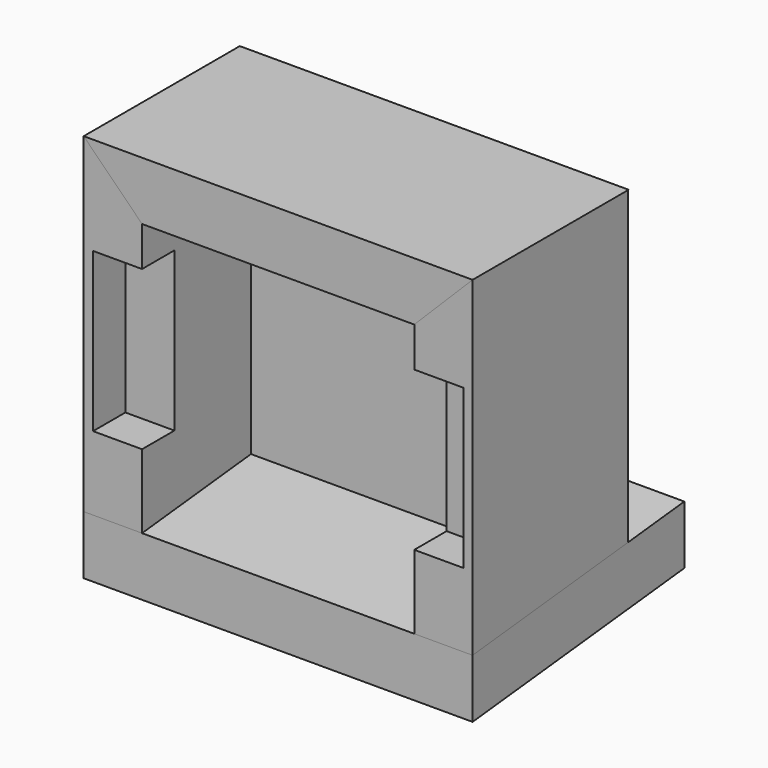
from build123d import *

# Parameters (mm, degrees)
F4_W        = 127
F4_H        = 103.27132
F5_DEPTH    = 19.05
F6_SIZE2    = 19.04999
F6_SIZE     = 19.04999
F7_SIZE2    = 2.002226
F7_SIZE     = 19.04999
F8_W        = 63.5
F8_H        = 107.95
F9_DEPTH    = 19.05
F10_SIZE2   = 6.674109
F10_SIZE    = 63.49999
F11_SIZE2   = 19.04999
F11_SIZE    = 19.04999
F12_W       = 63.5
F12_H       = 107.95
F13_DEPTH   = 19.05
F14_SIZE2   = 6.674109
F14_SIZE    = 63.49999
F15_SIZE2   = 19.04999
F15_SIZE    = 19.04999
F16_W       = 127
F16_H       = 63.7083128998
F17_DEPTH   = 19.05
F18_SIZE2   = 19.04999
F18_SIZE    = 19.04999
F20_W       = 127
F20_H       = 88.9
F21_DEPTH   = 19.05
F22_SIZE2   = 2.002226
F22_SIZE    = 19.04999
F22_2_SIZE2 = 2.002226
F22_2_SIZE  = 19.04999
F23_W       = 120.904
F23_H       = 51.816
F24_DEPTH   = 13.208


# Not quite as in the source:
# - a fillet or chamfer is up to 0.001 mm smaller than in the source, because OpenCascade refuses the exact size


with BuildPart() as f5:
    # F4 (on Front) → F5 (new body)
    with BuildSketch(Plane.XZ):
        with Locations((0, 11.86434)):
            Rectangle(F4_W, F4_H)
    extrude(amount=F5_DEPTH)

    # F6 (size 19.05 and 19.05 in the source; OpenCascade refuses exactly that, so slightly less here)
    f6_edges = [f5.edges().sort_by_distance(p)[0] for p in [
        (63.5, -19.05, 11.86434),
        (0, -19.05, 63.5),
        (-63.5, -19.05, 11.86434),
    ]]
    chamfer(f6_edges, length=F6_SIZE, length2=F6_SIZE2)

    # F7 (size 19.05 and 2.0022356818 in the source; OpenCascade refuses exactly that, so slightly less here)
    f7_edges = [f5.edges().sort_by_distance(p)[0] for p in [
        (0, 0, -39.77132),
    ]]
    f7_side = f5.faces().sort_by_distance((0, -8.964706, -39.77132))[0]
    chamfer(f7_edges, length=F7_SIZE, length2=F7_SIZE2, reference=f7_side)


with BuildPart() as f9:
    # F8 (on offset) → F9 (new body)
    with BuildSketch(Plane.YZ.offset(-63.5)):
        with Locations((-31.75, 9.525)):
            Rectangle(F8_W, F8_H)
    extrude(amount=F9_DEPTH)

    # F10 (size 63.5 and 6.6741189394 in the source; OpenCascade refuses exactly that, so slightly less here)
    f10_edges = [f9.edges().sort_by_distance(p)[0] for p in [
        (-53.975, 0, -44.45),
    ]]
    f10_side = f9.faces().sort_by_distance((-53.975, -31.75, -44.45))[0]
    chamfer(f10_edges, length=F10_SIZE, length2=F10_SIZE2, reference=f10_side)

    # F11 (size 19.05 and 19.05 in the source; OpenCascade refuses exactly that, so slightly less here)
    f11_edges = [f9.edges().sort_by_distance(p)[0] for p in [
        (-44.45, 0, 12.862054),
        (-44.45, -31.75, 63.5),
    ]]
    chamfer(f11_edges, length=F11_SIZE, length2=F11_SIZE2)


with BuildPart() as f13:
    # F12 (on offset) → F13 (new body)
    with BuildSketch(Plane.YZ.offset(63.5)):
        with Locations((-31.75, 9.525)):
            Rectangle(F12_W, F12_H)
    extrude(amount=-F13_DEPTH)

    # F14 (size 63.5 and 6.6741189394 in the source; OpenCascade refuses exactly that, so slightly less here)
    f14_edges = [f13.edges().sort_by_distance(p)[0] for p in [
        (53.975, 0, -44.45),
    ]]
    f14_side = f13.faces().sort_by_distance((53.975, -31.75, -44.45))[0]
    chamfer(f14_edges, length=F14_SIZE, length2=F14_SIZE2, reference=f14_side)

    # F15 (size 19.05 and 19.05 in the source; OpenCascade refuses exactly that, so slightly less here)
    f15_edges = [f13.edges().sort_by_distance(p)[0] for p in [
        (44.45, 0, 12.862054),
        (44.45, -31.75, 63.5),
    ]]
    chamfer(f15_edges, length=F15_SIZE, length2=F15_SIZE2)


with BuildPart() as f17:
    # F16 (on offset) → F17 (new body)
    with BuildSketch(Plane.XY.offset(63.5)):
        with Locations((0, -31.6458435501)):
            Rectangle(F16_W, F16_H)
    extrude(amount=-F17_DEPTH)

    # F18 (size 19.05 and 19.05 in the source; OpenCascade refuses exactly that, so slightly less here)
    f18_edges = [f17.edges().sort_by_distance(p)[0] for p in [
        (0, 0.208313, 44.45),
        (63.5, -31.645844, 44.45),
        (-63.5, -31.645844, 44.45),
    ]]
    chamfer(f18_edges, length=F18_SIZE, length2=F18_SIZE2)


with BuildPart() as f21:
    # F20 (on face) → F21 (new body)
    with BuildSketch(Plane(origin=(0, 3.9270236517, -37.3631342428), x_dir=(1, 0, 0), z_dir=(0, -0.1045284633, 0.9945218954))):
        with Locations((0, -25.3512205481)):
            Rectangle(F20_W, F20_H)
    extrude(amount=-F21_DEPTH)

    # F22 (size 19.05 and 2.0022356818 in the source; OpenCascade refuses exactly that, so slightly less here)
    f22_edges = [f21.edges().sort_by_distance(p)[0] for p in [
        (0, -65.491819, -44.659349),
    ]]
    f22_side = f21.faces().sort_by_distance((0, -64.496185, -54.13217))[0]
    chamfer(f22_edges, length=F22_SIZE, length2=F22_SIZE2, reference=f22_side)

    # F22#2 (size 19.05 and 2.0022356818 in the source; OpenCascade refuses exactly that, so slightly less here)
    f22_2_edges = [f21.edges().sort_by_distance(p)[0] for p in [
        (0, 24.912445, -54.31241),
    ]]
    f22_2_side = f21.faces().sort_by_distance((0, 23.916812, -44.839589))[0]
    chamfer(f22_2_edges, length=F22_2_SIZE, length2=F22_2_SIZE2, reference=f22_2_side)


with BuildPart() as f24:
    # F23 (on offset) → F24 (new body)
    with BuildSketch(Plane.XZ.offset(63.5)):
        with Locations((0, 5.588)):
            Rectangle(F23_W, F23_H)
    extrude(amount=-F24_DEPTH)


with BuildPart() as f13_1:
    add(f13.part)

    # F25: cut F24
    add(f24.part, mode=Mode.SUBTRACT)


with BuildPart() as f9_1:
    add(f9.part)

    # F25: cut F24
    add(f24.part, mode=Mode.SUBTRACT)


solid = Compound([f5.part, f17.part, f21.part, f13_1.part, f9_1.part])
